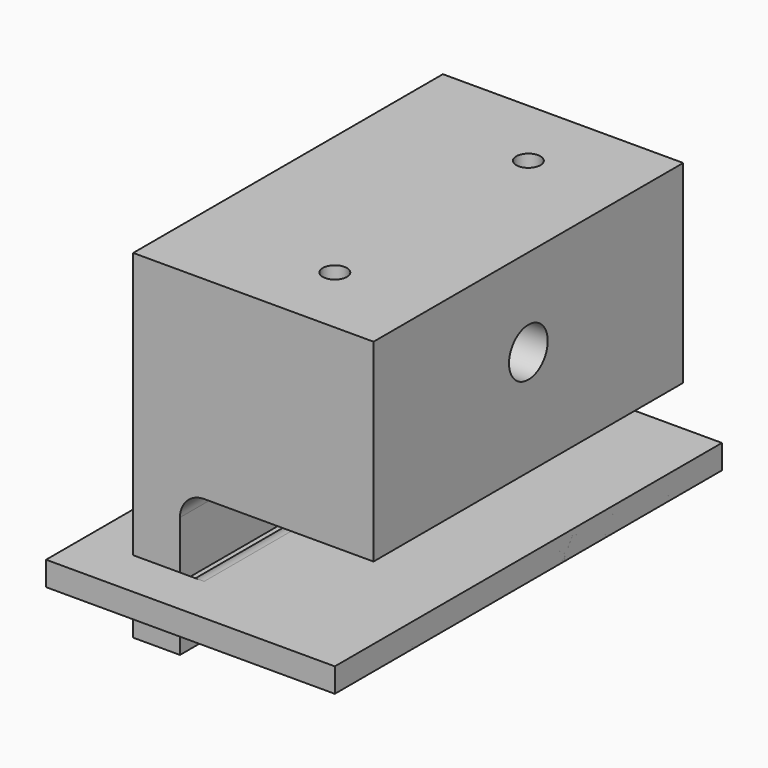
from build123d import *

# Parameters (mm, degrees)
F1_DEPTH  = 25.4
F3_D      = 6.35
F6_DEPTH  = 3.175
F7_D      = 3.175
F10_DEPTH = 2.54
F11_W     = 37.8906604153
F11_H     = 63.5
F11_W_2   = 6.1406604153
F11_H_2   = 50.8
F12_DEPTH = 3.175
F13_R     = 3.17499


# Not quite as in the source:
# - a fillet or chamfer is up to 0.001 mm smaller than in the source, because OpenCascade refuses the exact size


with BuildPart() as f1:
    # F0 (on Front) → F1 (new body, symmetric)
    with BuildSketch(Plane.XZ):
        with BuildLine():
            ThreePointArc((-7.5711545896, -3.175), (-6.6412186199, -0.9299359697), (-4.3961545896, 0))
            Line((-4.3961545896, 0), (17.8288454104, 0))
            Line((17.8288454104, 0), (17.8288454104, 25.4))
            Line((17.8288454104, 25.4), (-13.7118150049, 25.4))
            Line((-13.7118150049, 25.4), (-13.7118150049, -19.05))
            Line((-13.7118150049, -19.05), (-7.5711545896, -19.05))
            Line((-7.5711545896, -19.05), (-7.5711545896, -3.175))
        make_face()
    extrude(amount=F1_DEPTH, both=True)

    # F3 (through all)
    with Locations(Plane.YZ.offset(17.8288454104)):
        with Locations((0, 13.8620808721)):
            Hole(F3_D / 2)

    # F5 (on face) → F6 (cut)
    with BuildSketch(Plane(origin=(0, 0, 0), x_dir=(1, 0, 0), z_dir=(0, 0, -1))):
        Polygon((3.950722829, 10.5034171622), (9.1917113157, 12.1689244969), (10.3698338971, 17.5405073346), (6.3069679918, 21.2465828378), (1.065979505, 19.5810755031), (-0.1121430764, 14.2094926654), align=None)
        Polygon((0.7661597851, -19.2229619375), (5.8469226865, -21.327177549), (10.2096083118, -17.9792156115), (9.4915310357, -12.5270380625), (4.4107681342, -10.422822451), (0.048082509, -13.7707843885), align=None)
    extrude(amount=-F6_DEPTH, mode=Mode.SUBTRACT)

    # F7 (through all)
    with Locations(Plane(origin=(0, 0, 0), x_dir=(1, 0, 0), z_dir=(0, 0, -1))):
        with Locations((5.1288454104, -15.875), (5.1288454104, 15.875)):
            Hole(F7_D / 2)


with BuildPart() as f10:
    # F9 (on offset) → F10 (new body)
    with BuildSketch(Plane.XY.offset(-12.7)):
        with BuildLine():
            Line((17.8288454104, -31.75), (17.8288454104, 31.75))
            Line((17.8288454104, 31.75), (-13.7118150049, 31.75))
            Line((-13.7118150049, 31.75), (-13.7118150049, 26.035))
            Line((-13.7118150049, 26.035), (-7.5711545896, 26.035))
            ThreePointArc((-7.5711545896, 26.035), (-7.1221417836, 25.8490128061), (-6.9361545896, 25.4))
            Line((-6.9361545896, 25.4), (-6.9361545896, -25.4))
            ThreePointArc((-6.9361545896, -25.4), (-7.1221417836, -25.8490128061), (-7.5711545896, -26.035))
            Line((-7.5711545896, -26.035), (-13.7118150049, -26.035))
            Line((-13.7118150049, -26.035), (-13.7118150049, -31.75))
            Line((-13.7118150049, -31.75), (17.8288454104, -31.75))
        make_face()
    extrude(amount=F10_DEPTH)


with BuildPart() as f12:
    # F11 (on offset) → F12 (new body)
    with BuildSketch(Plane.XY.offset(-12.7)):
        with Locations((-1.1164847973, 0)):
            Rectangle(F11_W, F11_H)
        with Locations((-10.6414847973, 0)):
            Rectangle(F11_W_2, F11_H_2, mode=Mode.SUBTRACT)
    extrude(amount=F12_DEPTH)

    # F13 (radius 3.175 in the source; OpenCascade refuses exactly that, so slightly less here)
    f13_edges = [f12.edges().sort_by_distance(p)[0] for p in [
        (-7.571155, 0, -9.525),
    ]]
    fillet(f13_edges, radius=F13_R)


solid = Compound([f1.part, f10.part, f12.part])
